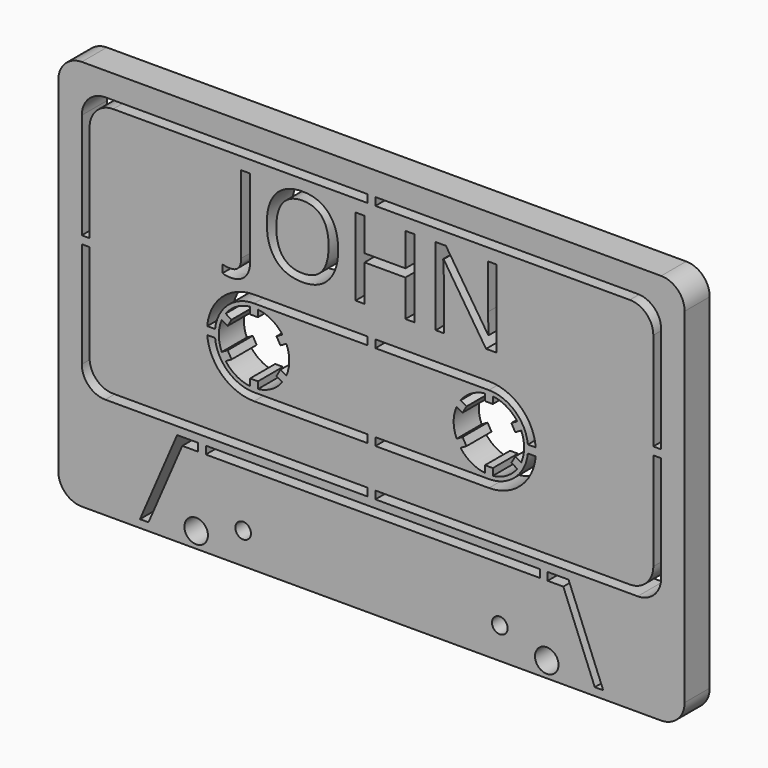
from build123d import *

# Parameters (mm, degrees)
F0_R         = 1.905
F0_R_2       = 1.27
F0_W         = 54.1864509355
F0_H         = 1.27
F1_DEPTH     = 5.08
F2_TEXT_SIZE = 17.6388888889
F3_DEPTH     = 25.4


# Not quite as in the source:
# - Text() gives the source's letters only with a copy of the font that has no kerning and outlines rounded to 1/6400 em; it was checked with that copy


with BuildPart() as f1:
    # F0 (on Front) → F1 (new body)
    with BuildSketch(Plane.XZ):
        with BuildLine():
            ThreePointArc((50.8, 27.94), (49.6840768363, 30.6340768363), (46.99, 31.75))
            Line((46.99, 31.75), (-46.99, 31.75))
            ThreePointArc((-46.99, 31.75), (-49.6840768363, 30.6340768363), (-50.8, 27.94))
            Line((-50.8, 27.94), (-50.8, -27.94))
            ThreePointArc((-50.8, -27.94), (-49.6840768363, -30.6340768363), (-46.99, -31.75))
            Line((-46.99, -31.75), (46.99, -31.75))
            ThreePointArc((46.99, -31.75), (49.6840768363, -30.6340768363), (50.8, -27.94))
            Line((50.8, -27.94), (50.8, 27.94))
        make_face()
        with Locations((-28.4354059759, -29.21)):
            Circle(F0_R, mode=Mode.SUBTRACT)
        Polygon((-36.1690502777, -30.48), (-37.5521693637, -30.48), (-31.5260323644, -16.51), (-28.1507439147, -16.51), (-28.1507439147, -17.78), (-30.6907439147, -17.78), align=None, mode=Mode.SUBTRACT)
        with Locations((-20.8154059759, -26.67)):
            Circle(F0_R_2, mode=Mode.SUBTRACT)
        with BuildLine():
            Line((-0.635, -15.24), (-43.18, -15.24))
            ThreePointArc((-43.18, -15.24), (-45.8740768363, -14.1240768363), (-46.99, -11.43))
            Line((-46.99, -11.43), (-46.99, 5.715))
            Line((-46.99, 5.715), (-45.72, 5.715))
            Line((-45.72, 5.715), (-45.72, -10.16))
            ThreePointArc((-45.72, -10.16), (-44.6040768363, -12.8540768363), (-41.91, -13.97))
            Line((-41.91, -13.97), (-0.635, -13.97))
            Line((-0.635, -13.97), (-0.635, -15.24))
        make_face(mode=Mode.SUBTRACT)
        with BuildLine():
            ThreePointArc((-25.3681702256, -0.635), (-23.3097094971, -4.7092860393), (-19.05, -6.35))
            Line((-19.05, -6.35), (-0.635, -6.35))
            Line((-0.635, -6.35), (-0.635, -7.62))
            Line((-0.635, -7.62), (-19.05, -7.62))
            ThreePointArc((-19.05, -7.62), (-24.2087643869, -5.6081681501), (-26.6434955719, -0.635))
            Line((-26.6434955719, -0.635), (-25.3681702256, -0.635))
        make_face(mode=Mode.SUBTRACT)
        with Locations((20.8154059759, -26.67)):
            Circle(F0_R_2, mode=Mode.SUBTRACT)
        with Locations((0.2124815531, -17.145)):
            Rectangle(F0_W, F0_H, mode=Mode.SUBTRACT)
        with Locations((28.4354059759, -29.21)):
            Circle(F0_R, mode=Mode.SUBTRACT)
        Polygon((28.5757070209, -16.51), (31.9739676356, -16.51), (37.589497303, -30.48), (36.2207339912, -30.48), (31.1157070209, -17.78), (28.5757070209, -17.78), align=None, mode=Mode.SUBTRACT)
        with BuildLine():
            Line((0.635, -7.62), (0.635, -6.35))
            Line((0.635, -6.35), (19.05, -6.35))
            ThreePointArc((19.05, -6.35), (23.3097094971, -4.7092860393), (25.3681702256, -0.635))
            Line((25.3681702256, -0.635), (26.6434955719, -0.635))
            ThreePointArc((26.6434955719, -0.635), (24.2087643869, -5.6081681501), (19.05, -7.62))
            Line((19.05, -7.62), (0.635, -7.62))
        make_face(mode=Mode.SUBTRACT)
        with BuildLine():
            ThreePointArc((46.99, -11.43), (45.8740768363, -14.1240768363), (43.18, -15.24))
            Line((43.18, -15.24), (0.635, -15.24))
            Line((0.635, -15.24), (0.635, -13.97))
            Line((0.635, -13.97), (41.91, -13.97))
            ThreePointArc((41.91, -13.97), (44.6040768363, -12.8540768363), (45.72, -10.16))
            Line((45.72, -10.16), (45.72, 5.715))
            Line((45.72, 5.715), (46.99, 5.715))
            Line((46.99, 5.715), (46.99, -11.43))
        make_face(mode=Mode.SUBTRACT)
        with BuildLine():
            ThreePointArc((-23.6511888497, 3.3897324628), (-21.9075, 4.9493351826), (-19.685, 5.6796126628))
            Line((-19.685, 5.6796126628), (-19.685, 4.572))
            Line((-19.685, 4.572), (-18.415, 4.572))
            Line((-18.415, 4.572), (-18.415, 5.6796126628))
            ThreePointArc((-18.415, 5.6796126628), (-16.1925, 4.9493351826), (-14.4488111503, 3.3897324628))
            Line((-14.4488111503, 3.3897324628), (-15.4080318539, 2.8359261314))
            Line((-15.4080318539, 2.8359261314), (-14.7730318539, 1.7360738686))
            Line((-14.7730318539, 1.7360738686), (-13.8138111503, 2.2898802))
            ThreePointArc((-13.8138111503, 2.2898802), (-13.335, 0), (-13.8138111503, -2.2898802))
            Line((-13.8138111503, -2.2898802), (-14.7730318539, -1.7360738686))
            Line((-14.7730318539, -1.7360738686), (-15.4080318539, -2.8359261314))
            Line((-15.4080318539, -2.8359261314), (-14.4488111503, -3.3897324628))
            ThreePointArc((-14.4488111503, -3.3897324628), (-16.1925, -4.9493351826), (-18.415, -5.6796126628))
            Line((-18.415, -5.6796126628), (-18.415, -4.572))
            Line((-18.415, -4.572), (-19.685, -4.572))
            Line((-19.685, -4.572), (-19.685, -5.6796126628))
            ThreePointArc((-19.685, -5.6796126628), (-21.9075, -4.9493351826), (-23.6511888497, -3.3897324628))
            Line((-23.6511888497, -3.3897324628), (-22.6919681461, -2.8359261314))
            Line((-22.6919681461, -2.8359261314), (-23.3269681461, -1.7360738686))
            Line((-23.3269681461, -1.7360738686), (-24.2861888497, -2.2898802))
            ThreePointArc((-24.2861888497, -2.2898802), (-24.765, 0), (-24.2861888497, 2.2898802))
            Line((-24.2861888497, 2.2898802), (-23.3269681461, 1.7360738686))
            Line((-23.3269681461, 1.7360738686), (-22.6919681461, 2.8359261314))
            Line((-22.6919681461, 2.8359261314), (-23.6511888497, 3.3897324628))
        make_face(mode=Mode.SUBTRACT)
        with BuildLine():
            Line((-0.635, 6.35), (-19.05, 6.35))
            ThreePointArc((-19.05, 6.35), (-23.3097094971, 4.7092860393), (-25.3681702256, 0.635))
            Line((-25.3681702256, 0.635), (-26.6434955719, 0.635))
            ThreePointArc((-26.6434955719, 0.635), (-24.2087643869, 5.6081681501), (-19.05, 7.62))
            Line((-19.05, 7.62), (-0.635, 7.62))
            Line((-0.635, 7.62), (-0.635, 6.35))
        make_face(mode=Mode.SUBTRACT)
        with BuildLine():
            ThreePointArc((-46.99, 24.13), (-45.8740768363, 26.8240768363), (-43.18, 27.94))
            Line((-43.18, 27.94), (-0.635, 27.94))
            Line((-0.635, 27.94), (-0.635, 26.67))
            Line((-0.635, 26.67), (-41.91, 26.67))
            ThreePointArc((-41.91, 26.67), (-44.6040768363, 25.5540768363), (-45.72, 22.86))
            Line((-45.72, 22.86), (-45.72, 6.985))
            Line((-45.72, 6.985), (-46.99, 6.985))
            Line((-46.99, 6.985), (-46.99, 24.13))
        make_face(mode=Mode.SUBTRACT)
        with BuildLine():
            ThreePointArc((14.4488111503, 3.3897324628), (16.1925, 4.9493351826), (18.415, 5.6796126628))
            Line((18.415, 5.6796126628), (18.415, 4.572))
            Line((18.415, 4.572), (19.685, 4.572))
            Line((19.685, 4.572), (19.685, 5.6796126628))
            ThreePointArc((19.685, 5.6796126628), (21.9075, 4.9493351826), (23.6511888497, 3.3897324628))
            Line((23.6511888497, 3.3897324628), (22.6919681461, 2.8359261314))
            Line((22.6919681461, 2.8359261314), (23.3269681461, 1.7360738686))
            Line((23.3269681461, 1.7360738686), (24.2861888497, 2.2898802))
            ThreePointArc((24.2861888497, 2.2898802), (24.765, 0), (24.2861888497, -2.2898802))
            Line((24.2861888497, -2.2898802), (23.3269681461, -1.7360738686))
            Line((23.3269681461, -1.7360738686), (22.6919681461, -2.8359261314))
            Line((22.6919681461, -2.8359261314), (23.6511888497, -3.3897324628))
            ThreePointArc((23.6511888497, -3.3897324628), (21.9075, -4.9493351826), (19.685, -5.6796126628))
            Line((19.685, -5.6796126628), (19.685, -4.572))
            Line((19.685, -4.572), (18.415, -4.572))
            Line((18.415, -4.572), (18.415, -5.6796126628))
            ThreePointArc((18.415, -5.6796126628), (16.1925, -4.9493351826), (14.4488111503, -3.3897324628))
            Line((14.4488111503, -3.3897324628), (15.4080318539, -2.8359261314))
            Line((15.4080318539, -2.8359261314), (14.7730318539, -1.7360738686))
            Line((14.7730318539, -1.7360738686), (13.8138111503, -2.2898802))
            ThreePointArc((13.8138111503, -2.2898802), (13.335, 0), (13.8138111503, 2.2898802))
            Line((13.8138111503, 2.2898802), (14.7730318539, 1.7360738686))
            Line((14.7730318539, 1.7360738686), (15.4080318539, 2.8359261314))
            Line((15.4080318539, 2.8359261314), (14.4488111503, 3.3897324628))
        make_face(mode=Mode.SUBTRACT)
        with BuildLine():
            Line((0.635, 6.35), (0.635, 7.62))
            Line((0.635, 7.62), (19.05, 7.62))
            ThreePointArc((19.05, 7.62), (21.2497045256, 7.2955945611), (23.2621134838, 6.35))
            ThreePointArc((23.2621134838, 6.35), (25.6080795622, 3.880205208), (26.6434955719, 0.635))
            Line((26.6434955719, 0.635), (25.3681702256, 0.635))
            ThreePointArc((25.3681702256, 0.635), (23.3097094971, 4.7092860393), (19.05, 6.35))
            Line((19.05, 6.35), (0.635, 6.35))
        make_face(mode=Mode.SUBTRACT)
        with BuildLine():
            ThreePointArc((43.18, 27.94), (45.8740768363, 26.8240768363), (46.99, 24.13))
            Line((46.99, 24.13), (46.99, 6.985))
            Line((46.99, 6.985), (45.72, 6.985))
            Line((45.72, 6.985), (45.72, 22.86))
            ThreePointArc((45.72, 22.86), (44.6040768363, 25.5540768363), (41.91, 26.67))
            Line((41.91, 26.67), (0.635, 26.67))
            Line((0.635, 26.67), (0.635, 27.94))
            Line((0.635, 27.94), (43.18, 27.94))
        make_face(mode=Mode.SUBTRACT)
    extrude(amount=F1_DEPTH)

    # F2 (on face) → F3 (cut)
    with BuildSketch(Plane.XZ.offset(5.08)):
        with Locations((-22.7711, 12.1012137619)):
            Text('JOHN', F2_TEXT_SIZE, font='Open Sans', text_align=(TextAlign.LEFT, TextAlign.BOTTOM))
    extrude(amount=-F3_DEPTH, mode=Mode.SUBTRACT)


solid = f1.part
